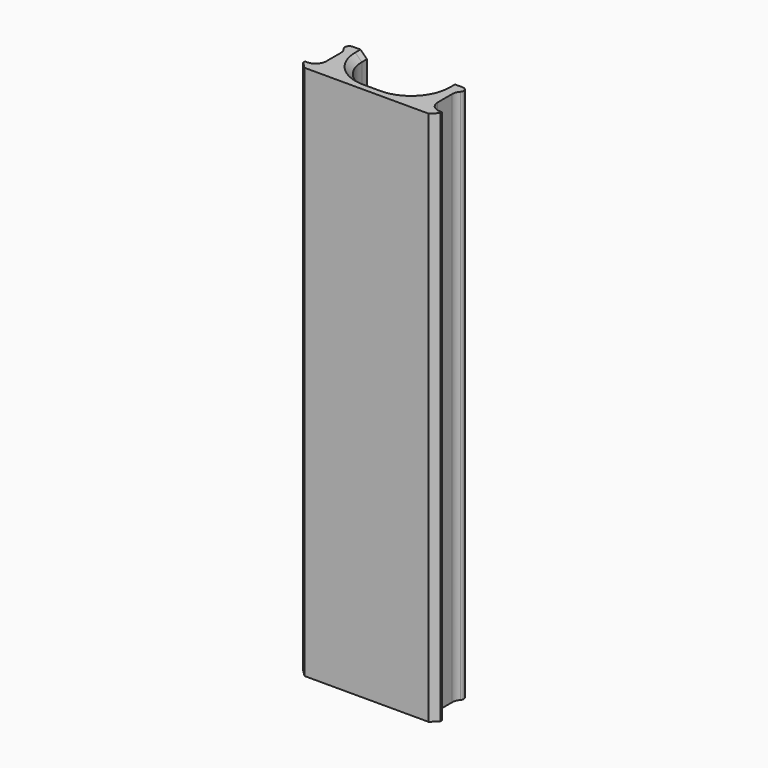
from build123d import *

# Parameters (mm, degrees)
F1_DEPTH    = 25
F2_T1_DEPTH = 25
F3_R        = 0.5
F4_T1_DEPTH = 26.7320508076
F5_R        = 0.2
F6_W        = 3.8095204468
F6_H        = 1.8
F7_DEPTH    = 25.0010001
F8_R        = 1.5
F9_SIZE     = 0.3


# Not quite as in the source:
# - a fillet or chamfer that OpenCascade refuses, or shapes differently, is made with other operations: its cross-section is extruded or revolved along the edge and cut away or added


with BuildPart() as f1:
    # F0 (on Top) → F1 (new body)
    with BuildSketch(Plane.XY):
        Polygon((0, 0.4), (0, 0), (6.4, 0), (6.4, 0.4), (5.8, 0.4), (5.8, 2.2), (6.1, 2.2), (6.1, 2.4), (0.3, 2.4), (0.3, 2.2), (0.6, 2.2), (0.6, 0.4), align=None)
    extrude(amount=F1_DEPTH)

    # F2: fillet of radius 0.5 on 2 edges, made by hand

    # F2_s2 → F2_t1 (join)
    with BuildSketch(Plane.XY):
        with BuildLine():
            ThreePointArc((0.3, 2.2), (0.5183300133, 2.0156037093), (0.6, 1.7417424305))
            Line((0.6, 1.7417424305), (0.6, 2.2))
            Line((0.6, 2.2), (0.3, 2.2))
        make_face()
        with BuildLine():
            ThreePointArc((5.8, 1.7417424305), (5.8816699867, 2.0156037093), (6.1, 2.2))
            Line((6.1, 2.2), (5.8, 2.2))
            Line((5.8, 2.2), (5.8, 1.7417424305))
        make_face()
    extrude(amount=F2_T1_DEPTH)

    # F3
    f3_edges = [f1.edges().sort_by_distance(p)[0] for p in [
        (5.8, 0.4, 12.5),
        (0.6, 0.4, 12.5),
    ]]
    fillet(f3_edges, radius=F3_R)

    # F4: fillet of radius 0.4 on 2 edges, made by hand

    # F4_s2 → F4_t1 (cut)
    with BuildSketch(Plane.XY.offset(-0.8660254038)):
        with BuildLine():
            ThreePointArc((0.3, 2.2), (0.4464101615, 2.3464101615), (0.6464101615, 2.4))
            Line((0.6464101615, 2.4), (0.3, 2.4))
            Line((0.3, 2.4), (0.3, 2.2))
        make_face()
        with BuildLine():
            ThreePointArc((5.7535898385, 2.4), (5.9535898385, 2.3464101615), (6.1, 2.2))
            Line((6.1, 2.2), (6.1, 2.4))
            Line((6.1, 2.4), (5.7535898385, 2.4))
        make_face()
    extrude(amount=F4_T1_DEPTH, mode=Mode.SUBTRACT)

    # F5
    f5_edges = [f1.edges().sort_by_distance(p)[0] for p in [
        (0.3, 2.2, 12.5),
        (6.1, 2.2, 12.5),
    ]]
    fillet(f5_edges, radius=F5_R)

    # F6 (on face) → F7 (cut, through all)
    with BuildSketch(Plane.XY.offset(25)):
        with Locations((3.2, 1.5)):
            Rectangle(F6_W, F6_H)
    extrude(amount=-F7_DEPTH, mode=Mode.SUBTRACT)

    # F8
    f8_edges = [f1.edges().sort_by_distance(p)[0] for p in [
        (1.29524, 0.6, 12.5),
        (5.10476, 0.6, 12.5),
    ]]
    fillet(f8_edges, radius=F8_R)

    # F9
    f9_edges = [f1.edges().sort_by_distance(p)[0] for p in [
        (3.2, 0.6, 25),
        (2.79524, 0.6, 12.5),
        (3.60476, 0.6, 12.5),
        (3.2, 0.6, 0),
        (6.4, 0, 12.5),
        (0, 0, 12.5),
        (1.29524, 2.25, 0),
        (1.73458, 1.03934, 0),
        (4.66542, 1.03934, 0),
        (5.10476, 2.25, 0),
        (1.29524, 2.25, 25),
        (1.73458, 1.03934, 25),
        (4.66542, 1.03934, 25),
        (5.10476, 2.25, 25),
    ]]
    chamfer(f9_edges, length=F9_SIZE)


solid = f1.part
